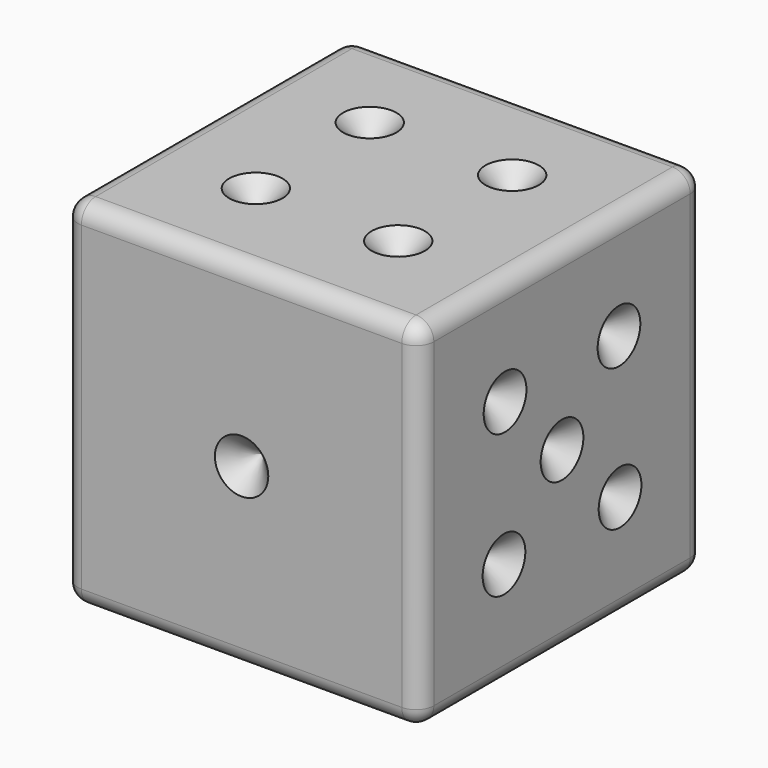
from build123d import *

# Parameters (mm, degrees)
F0_W      = 20
F0_H      = 20
F1_DEPTH  = 20
F2_R      = 1.5
F3_DEPTH  = 1.5
F4_R      = 1
F5_R      = 1.5
F6_DEPTH  = 1.5
F7_R      = 1.5
F8_DEPTH  = 1.5
F9_R      = 1.5
F10_DEPTH = 1.5
F11_R     = 1.5
F12_DEPTH = 1.5
F13_R     = 1.5
F14_DEPTH = 1.5
F15_SIZE  = 1.49999


# Not quite as in the source:
# - a fillet or chamfer is up to 0.001 mm smaller than in the source, because OpenCascade refuses the exact size


with BuildPart() as f1:
    # F0 (on Top) → F1 (new body)
    with BuildSketch(Plane.XY):
        with Locations((10, 10)):
            Rectangle(F0_W, F0_H)
    extrude(amount=F1_DEPTH)

    # F2 (on face) → F3 (cut)
    with BuildSketch(Plane.XZ):
        with Locations((10, 10)):
            Circle(F2_R)
    extrude(amount=-F3_DEPTH, mode=Mode.SUBTRACT)

    # F4
    f4_edges = [f1.edges().sort_by_distance(p)[0] for p in [
        (0, 10, 20),
        (10, 20, 20),
        (20, 10, 20),
        (10, 0, 20),
        (20, 0, 10),
        (10, 0, 0),
        (0, 0, 10),
        (20, 10, 0),
        (20, 20, 10),
        (10, 20, 0),
        (0, 10, 0),
        (0, 20, 10),
    ]]
    fillet(f4_edges, radius=F4_R)

    # F5 (on face) → F6 (cut)
    with BuildSketch(Plane.XY.offset(20)):
        with Locations((6, 14)):
            Circle(F5_R)
        with Locations((6, 6)):
            Circle(F5_R)
        with Locations((14, 6)):
            Circle(F5_R)
        with Locations((14, 14)):
            Circle(F5_R)
    extrude(amount=-F6_DEPTH, mode=Mode.SUBTRACT)

    # F7 (on face) → F8 (cut)
    with BuildSketch(Plane.YZ.offset(20)):
        with Locations((6, 14)):
            Circle(F7_R)
        with Locations((5.9253086879, 5.9995350826)):
            Circle(F7_R)
        with Locations((10, 10)):
            Circle(F7_R)
        with Locations((14, 14)):
            Circle(F7_R)
        with Locations((14.0746913121, 5.9995350826)):
            Circle(F7_R)
    extrude(amount=-F8_DEPTH, mode=Mode.SUBTRACT)

    # F9 (on face) → F10 (cut)
    with BuildSketch(Plane(origin=(0, 0, 0), x_dir=(1, 0, 0), z_dir=(0, 0, -1))):
        with Locations((5.1866916474, -5.1866916474)):
            Circle(F9_R)
        with Locations((10, -10)):
            Circle(F9_R)
        with Locations((15.44734044, -15.44734044)):
            Circle(F9_R)
    extrude(amount=-F10_DEPTH, mode=Mode.SUBTRACT)

    # F11 (on face) → F12 (cut)
    with BuildSketch(Plane(origin=(0, 20, 0), x_dir=(-1, 0, 0), z_dir=(0, 1, 0))):
        with Locations((-14, 15.0308646262)):
            Circle(F11_R)
        with Locations((-14, 10)):
            Circle(F11_R)
        with Locations((-14.1852116212, 4.5415428467)):
            Circle(F11_R)
        with Locations((-5.8147883788, 4.5415428467)):
            Circle(F11_R)
        with Locations((-6, 10)):
            Circle(F11_R)
        with Locations((-6, 15.0308646262)):
            Circle(F11_R)
    extrude(amount=-F12_DEPTH, mode=Mode.SUBTRACT)

    # F13 (on face) → F14 (cut)
    with BuildSketch(Plane(origin=(0, 0, 0), x_dir=(0, -1, 0), z_dir=(-1, 0, 0))):
        with Locations((-10, 6.2473174185)):
            Circle(F13_R)
        with Locations((-10, 12.9042267799)):
            Circle(F13_R)
    extrude(amount=-F14_DEPTH, mode=Mode.SUBTRACT)

    # F15 (size 1.5 in the source; OpenCascade refuses exactly that, so slightly less here)
    f15_edges = [f1.edges().sort_by_distance(p)[0] for p in [
        (12.5, 14, 18.5),
        (12.5, 6, 18.5),
        (4.5, 6, 18.5),
        (4.5, 14, 18.5),
        (8.5, 1.5, 10),
        (18.5, 8.5, 10),
        (18.5, 4.5, 14),
        (18.5, 12.5, 14),
        (18.5, 12.574691, 5.999535),
        (18.5, 4.425309, 5.999535),
        (3.686692, 5.186692, 1.5),
        (8.5, 10, 1.5),
        (13.94734, 15.44734, 1.5),
        (15.5, 18.5, 15.030865),
        (7.5, 18.5, 15.030865),
        (15.5, 18.5, 10),
        (7.5, 18.5, 10),
        (15.685212, 18.5, 4.541543),
        (7.314788, 18.5, 4.541543),
        (1.5, 11.5, 6.247317),
        (1.5, 11.5, 12.904227),
    ]]
    chamfer(f15_edges, length=F15_SIZE)


solid = f1.part
